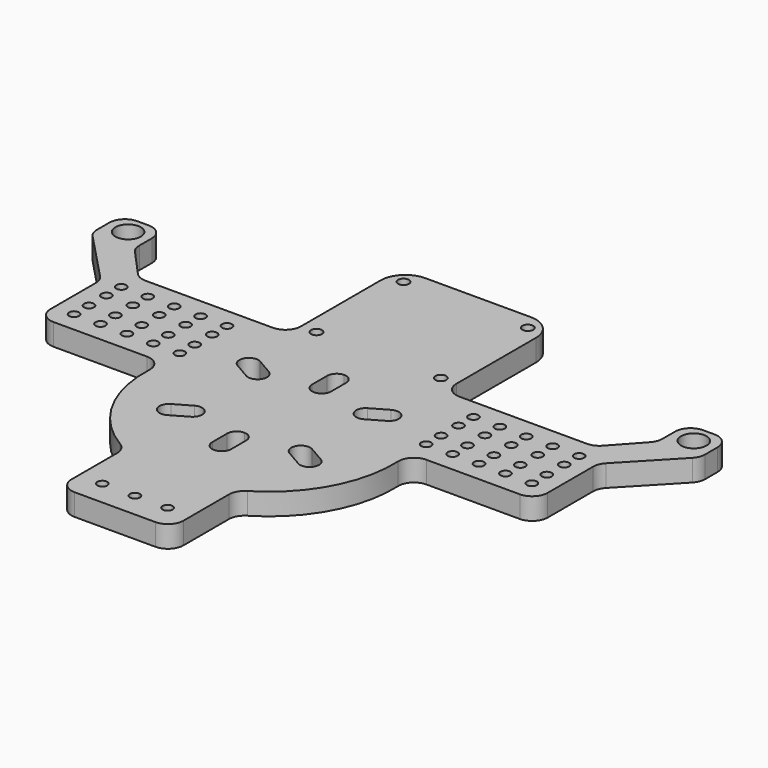
from build123d import *

# Parameters (mm, degrees)
F0_R     = 1.6
F0_R_2   = 4.1
F0_R_3   = 1.75
F1_DEPTH = 7
F2_R     = 5
F5_R     = 8
F0_W     = 19.9004877359
F0_H     = 28.2499268651
F6_DEPTH = 2.5


# Not quite as in the source:
# - two fillets or chamfers of one size are made in one step
# - a feature names something its author has since deleted; it is built from what else it names


with BuildPart() as f1:
    # F0 (on Top) → F1 (new body)
    with BuildSketch(Plane.XY):
        with BuildLine():
            Line((-80, 31.2532794885), (-80, 6))
            Line((-80, 6), (-39.382737335, 6))
            ThreePointArc((-39.382737335, 6), (-35.7696607995, -18.9033897988), (-18, -36.721142199))
            Line((-18, -36.721142199), (-18, -63))
            Line((-18, -63), (0, -63))
            Line((0, -63), (0, -56.6))
            ThreePointArc((0, -56.6), (-1.6, -55), (0, -53.4))
            Line((0, -53.4), (0, -23.1440107676))
            ThreePointArc((0, -23.1440107676), (-2.1566756826, -22.2506864502), (-3.05, -20.0940107676))
            Line((-3.05, -20.0940107676), (-3.05, -14.0940107676))
            ThreePointArc((-3.05, -14.0940107676), (-2.1566756826, -11.937335085), (0, -11.0440107676))
            Line((0, -11.0440107676), (0, 17.0440107676))
            ThreePointArc((0, 17.0440107676), (-2.1566756826, 17.937335085), (-3.05, 20.0940107676))
            Line((-3.05, 20.0940107676), (-3.05, 26.0940107676))
            ThreePointArc((-3.05, 26.0940107676), (-2.1566756826, 28.2506864502), (0, 29.1440107676))
            Line((0, 29.1440107676), (0, 38))
            Line((0, 38), (0, 46.1897078156))
            Line((0, 46.1897078156), (-19.9004877359, 46.1897078156))
            Line((-19.9004877359, 46.1897078156), (-19.9004877359, 74.4396346807))
            Line((-19.9004877359, 74.4396346807), (0, 74.4396346807))
            Line((0, 74.4396346807), (0, 83))
            Line((0, 83), (-25, 83))
            Line((-25, 83), (-25, 38))
            Line((-25, 38), (-73.253, 38))
            Line((-73.253, 38), (-84.158, 50))
            Line((-84.158, 50), (-84.158, 62))
            Line((-84.158, 62), (-97.842, 62))
            Line((-97.842, 62), (-97.842, 50))
            Line((-97.842, 50), (-80, 31.2532794885))
        make_face()
        with Locations((-10.5, -55)):
            Circle(F0_R, mode=Mode.SUBTRACT)
        with BuildLine():
            ThreePointArc((-21.0730762114, -15.6883828653), (-25.2394536929, -14.5720053838), (-24.1230762114, -10.4056279022))
            Line((-24.1230762114, -10.4056279022), (-18.9269237886, -7.4056279022))
            ThreePointArc((-18.9269237886, -7.4056279022), (-14.7605463071, -8.5220053838), (-15.8769237886, -12.6883828653))
            Line((-15.8769237886, -12.6883828653), (-21.0730762114, -15.6883828653))
        make_face(mode=Mode.SUBTRACT)
        with Locations((-73.6379495263, 12.566276442)):
            Circle(F0_R, mode=Mode.SUBTRACT)
        with Locations((-73.6379495263, 18.566276442)):
            Circle(F0_R, mode=Mode.SUBTRACT)
        with Locations((-73.6379495263, 25.566276442)):
            Circle(F0_R, mode=Mode.SUBTRACT)
        with Locations((-73.6379495263, 31.566276442)):
            Circle(F0_R, mode=Mode.SUBTRACT)
        with Locations((-65.1379495263, 12.566276442)):
            Circle(F0_R, mode=Mode.SUBTRACT)
        with Locations((-65.1379495263, 18.566276442)):
            Circle(F0_R, mode=Mode.SUBTRACT)
        with Locations((-56.6379495263, 12.566276442)):
            Circle(F0_R, mode=Mode.SUBTRACT)
        with Locations((-56.6379495263, 18.566276442)):
            Circle(F0_R, mode=Mode.SUBTRACT)
        with Locations((-65.1379495263, 25.566276442)):
            Circle(F0_R, mode=Mode.SUBTRACT)
        with Locations((-56.6379495263, 25.566276442)):
            Circle(F0_R, mode=Mode.SUBTRACT)
        with Locations((-48.1379495263, 12.566276442)):
            Circle(F0_R, mode=Mode.SUBTRACT)
        with Locations((-48.1379495263, 18.566276442)):
            Circle(F0_R, mode=Mode.SUBTRACT)
        with Locations((-39.6379495263, 12.566276442)):
            Circle(F0_R, mode=Mode.SUBTRACT)
        with Locations((-39.6379495263, 18.566276442)):
            Circle(F0_R, mode=Mode.SUBTRACT)
        with Locations((-48.1379495263, 25.566276442)):
            Circle(F0_R, mode=Mode.SUBTRACT)
        with Locations((-39.6379495263, 25.566276442)):
            Circle(F0_R, mode=Mode.SUBTRACT)
        with Locations((-65.1379495263, 31.566276442)):
            Circle(F0_R, mode=Mode.SUBTRACT)
        with Locations((-56.6379495263, 31.566276442)):
            Circle(F0_R, mode=Mode.SUBTRACT)
        with Locations((-48.1379495263, 31.566276442)):
            Circle(F0_R, mode=Mode.SUBTRACT)
        with Locations((-39.6379495263, 31.566276442)):
            Circle(F0_R, mode=Mode.SUBTRACT)
        with Locations((-91, 56)):
            Circle(F0_R_2, mode=Mode.SUBTRACT)
        with BuildLine():
            Line((-18.9269237886, 13.4056279022), (-24.1230762114, 16.4056279022))
            ThreePointArc((-24.1230762114, 16.4056279022), (-25.2394536929, 20.5720053838), (-21.0730762114, 21.6883828653))
            Line((-21.0730762114, 21.6883828653), (-15.8769237886, 18.6883828653))
            ThreePointArc((-15.8769237886, 18.6883828653), (-14.7605463071, 14.5220053838), (-18.9269237886, 13.4056279022))
        make_face(mode=Mode.SUBTRACT)
        with Locations((-20, 43)):
            Circle(F0_R_3, mode=Mode.SUBTRACT)
        with Locations((-20, 78)):
            Circle(F0_R_3, mode=Mode.SUBTRACT)
    extrude(amount=-F1_DEPTH)

    # F2
    f2_edges = [f1.edges().sort_by_distance(p)[0] for p in [
        (-39.382737, 6, -3.5),
        (-80, 6, -3.5),
        (-18, -36.721142, -3.5),
        (-18, -63, -3.5),
        (-73.253, 38, -3.5),
        (-84.158, 50, -3.5),
        (-84.158, 62, -3.5),
        (-97.842, 62, -3.5),
        (-97.842, 50, -3.5),
        (-80, 31.253279, -3.5),
        (-25, 38, -3.5),
    ]]
    fillet(f2_edges, radius=F2_R)

    # F3: F1 across plane


with BuildPart() as f1_1:
    add(f1.part)
    add(f1.part.mirror(Plane.YZ))

    # F5
    f5_edges = [f1_1.edges().sort_by_distance(p)[0] for p in [
        (-25, 83, -3.5),
        (25, 83, -3.5),
    ]]
    fillet(f5_edges, radius=F5_R)

    # F0 (on Top) → F6 (join)
    with BuildSketch(Plane.XY):
        with Locations((9.9502438679, 60.3146712482)):
            Rectangle(F0_W, F0_H)
        with Locations((-9.9502438679, 60.3146712482)):
            Rectangle(F0_W, F0_H)
    extrude(amount=-F6_DEPTH)


solid = f1_1.part
